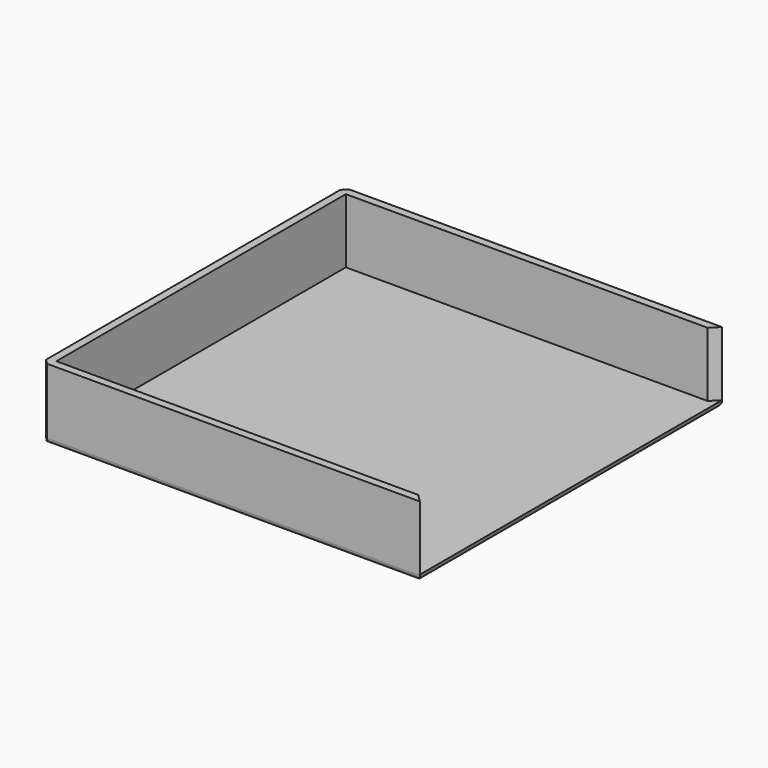
from build123d import *

# Parameters (mm, degrees)
F1_DEPTH    = 13
F2_W        = 76.2
F2_H        = 76.2
F3_DEPTH    = 1.2
F4_R        = 1
F5_T1_DEPTH = 18.3433659759


# Not quite as in the source:
# - a fillet or chamfer that OpenCascade refuses, or shapes differently, is made with other operations: its cross-section is extruded or revolved along the edge and cut away or added


with BuildPart() as f1:
    # F0 (on Top) → F1 (new body)
    with BuildSketch(Plane.XY):
        Polygon((-36.5, 36.5), (36.5, 36.5), (38.1, 38.1), (-38.1, 38.1), (-38.1, -38.1), (38.1, -38.1), (36.5, -36.5), (-36.5, -36.5), align=None)
    extrude(amount=F1_DEPTH)

    # F2 (on Top) → F3 (join)
    with BuildSketch(Plane.XY):
        Rectangle(F2_W, F2_H)
    extrude(amount=-F3_DEPTH)

    # F4
    f4_edges = [f1.edges().sort_by_distance(p)[0] for p in [
        (0, -38.1, -1.2),
        (38.1, 0, -1.2),
        (0, 38.1, -1.2),
        (-38.1, 0, -1.2),
    ]]
    fillet(f4_edges, radius=F4_R)

    # F5: chamfer of 1 on 2 edges, made by hand

    # F5_s2 → F5_t1 (cut)
    with BuildSketch(Plane.XY.offset(-2.771682988)):
        Polygon((-37.1, -38.1), (-38.1, -37.1), (-38.1, -38.1), align=None)
        Polygon((-38.1, 37.1), (-37.1, 38.1), (-38.1, 38.1), align=None)
    extrude(amount=F5_T1_DEPTH, mode=Mode.SUBTRACT)


solid = f1.part
